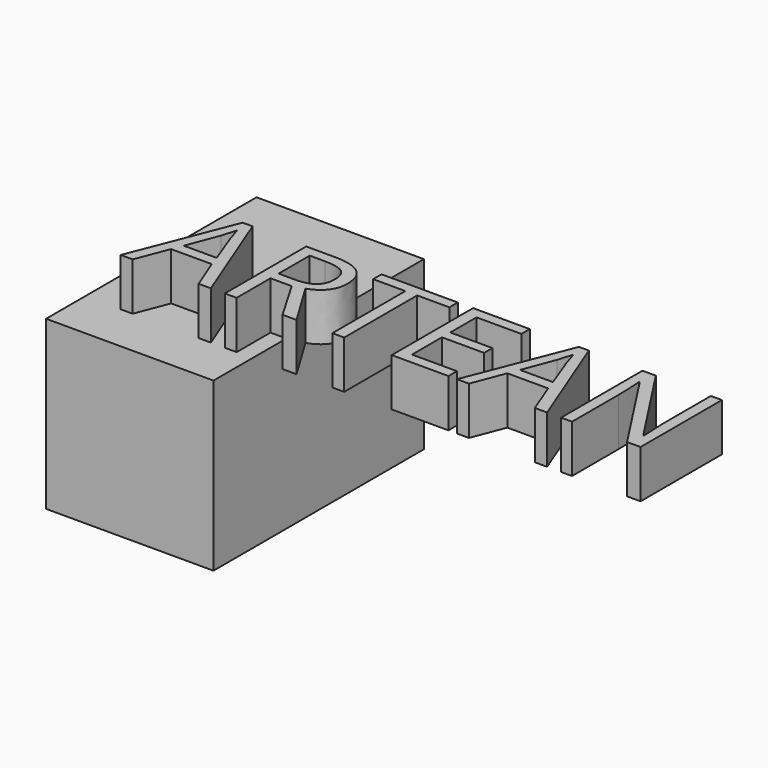
from build123d import *

# Parameters (mm, degrees)
F0_W         = 88.9
F0_H         = 88.9
F1_DEPTH     = 139.7
F2_TEXT_SIZE = 75.6635330617
F3_DEPTH     = 25.4


# Not quite as in the source:
# - Text() gives the source's letters only with a copy of the font that has no kerning and outlines rounded to 1/6400 em; it was checked with that copy


with BuildPart() as f1:
    # F0 (on Front) → F1 (new body)
    with BuildSketch(Plane.XZ):
        with Locations((27.7344211221, 34.5825339451)):
            Rectangle(F0_W, F0_H)
    extrude(amount=F1_DEPTH)

    # F2 (on face) → F3 (join)
    with BuildSketch(Plane.XY.offset(79.0325339451)):
        with Locations((2.1519688889, -113.7450709939)):
            Text('ARTEAN', F2_TEXT_SIZE, font='Open Sans', text_align=(TextAlign.LEFT, TextAlign.BOTTOM))
    extrude(amount=F3_DEPTH)


solid = f1.part
